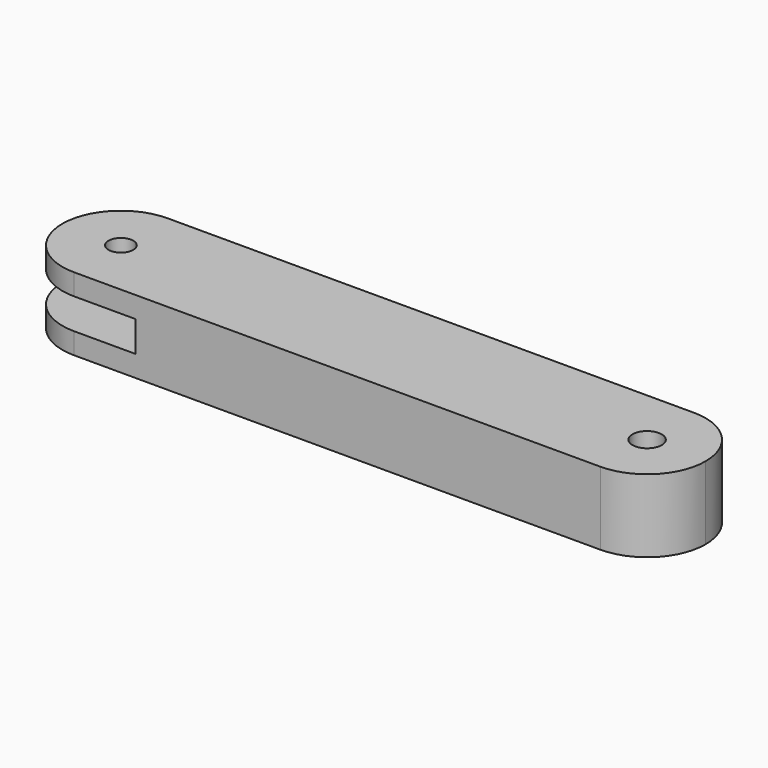
from build123d import *

# Parameters (mm, degrees)
F0_W     = 220
F0_H     = 40
F1_DEPTH = 12.5
F2_W     = 41
F2_H     = 10.5
F3_DEPTH = 20
F4_R     = 19.99999
F6_D     = 8.5
F8_D     = 10
F9_R     = 19.99999


# Not quite as in the source:
# - a fillet or chamfer is up to 0.001 mm smaller than in the source, because OpenCascade refuses the exact size


with BuildPart() as f1:
    # F0 (on Top) → F1 (new body, symmetric)
    with BuildSketch(Plane.XY):
        Rectangle(F0_W, F0_H)
    extrude(amount=F1_DEPTH, both=True)

    # F2 (on Front) → F3 (cut, symmetric)
    with BuildSketch(Plane.XZ):
        with Locations((-89.5, 0)):
            Rectangle(F2_W, F2_H)
    extrude(amount=F3_DEPTH, both=True, mode=Mode.SUBTRACT)

    # F4 (radius 20 in the source; OpenCascade refuses exactly that, so slightly less here)
    f4_edges = [f1.edges().sort_by_distance(p)[0] for p in [
        (-110, 20, 8.875),
        (-110, -20, 8.875),
        (-110, -20, -8.875),
        (-110, 20, -8.875),
    ]]
    fillet(f4_edges, radius=F4_R)

    # F6 (through all)
    with Locations(Plane(origin=(0, 0, -12.5), x_dir=(1, 0, 0), z_dir=(0, 0, -1))):
        with Locations((-90, 0)):
            Hole(F6_D / 2)

    # F8 (through all)
    with Locations(Plane(origin=(0, 0, -12.5), x_dir=(1, 0, 0), z_dir=(0, 0, -1))):
        with Locations((90, 0)):
            Hole(F8_D / 2)

    # F9 (radius 20 in the source; OpenCascade refuses exactly that, so slightly less here)
    f9_edges = [f1.edges().sort_by_distance(p)[0] for p in [
        (110, -20, 0),
        (110, 20, 0),
    ]]
    fillet(f9_edges, radius=F9_R)


solid = f1.part
